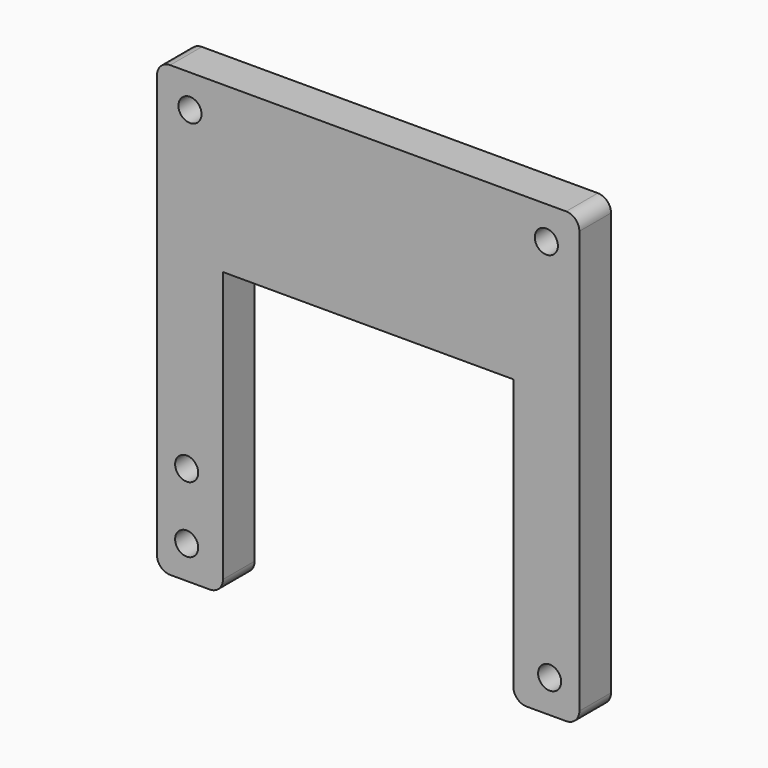
from build123d import *

# Parameters (mm, degrees)
F0_W     = 64
F0_H     = 68
F1_DEPTH = 6
F2_R     = 1.75
F3_DEPTH = 25
F4_R     = 2


# Not quite as in the source:
# - a feature names something its author has since deleted; it is built from what else it names


with BuildPart() as f1:
    # F0 (on Front) → F1 (new body)
    with BuildSketch(Plane.XZ):
        Rectangle(F0_W, F0_H)
    extrude(amount=F1_DEPTH)

    # F2 (on face) → F3 (cut)
    with BuildSketch(Plane.XZ.offset(6)):
        Polygon((22, 9), (0, 9), (-22, 9), (-22, -34), (22, -34), align=None)
        with Locations((27.5, -29)):
            Circle(F2_R)
        with Locations((-27.5, -19)):
            Circle(F2_R)
        with Locations((-27.5, -29)):
            Circle(F2_R)
        with Locations((-27, 29)):
            Circle(F2_R)
        with Locations((27, 29)):
            Circle(F2_R)
    extrude(amount=-F3_DEPTH, mode=Mode.SUBTRACT)

    # F4
    f4_edges = [f1.edges().sort_by_distance(p)[0] for p in [
        (-32, -3, 34),
        (32, -3, 34),
        (-32, -3, -34),
        (32, -3, -34),
        (-22, -3, -34),
        (22, -3, -34),
    ]]
    fillet(f4_edges, radius=F4_R)


solid = f1.part
